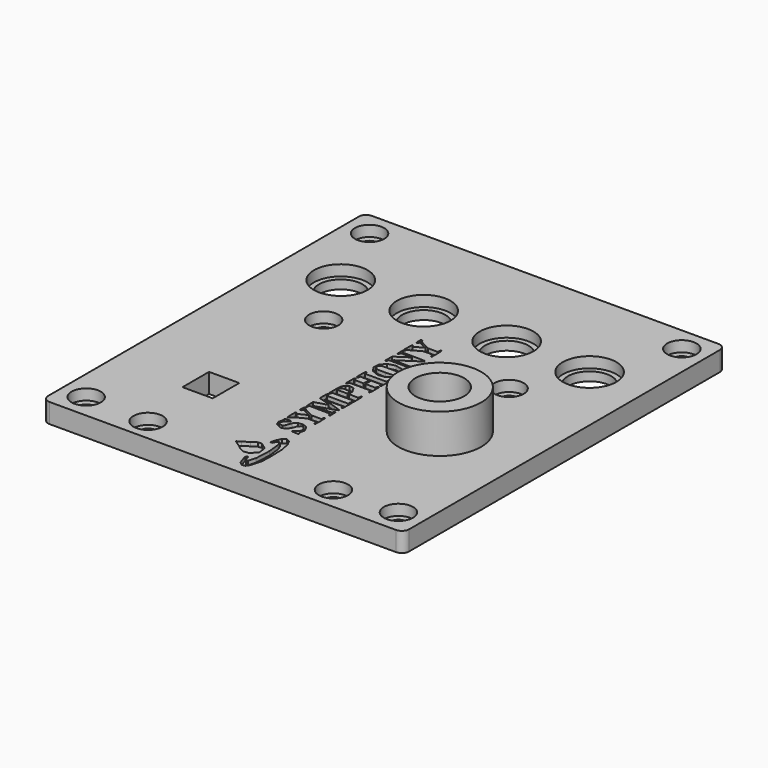
from build123d import *

# Parameters (mm, degrees)
F1_R      = 3
F1_R_2    = 1.75
F1_R_3    = 8.5
F1_R_4    = 0.9
F1_R_5    = 4.45
F1_R_6    = 1.7
F1_R_7    = 5
F1_W      = 7
F1_H      = 4.5
F2_DEPTH  = 4
F3_R      = 1.5
F4_R      = 3
F5_DEPTH  = 2.2
F6_R      = 5.5
F6_R_2    = 4.45
F7_DEPTH  = 2.2
F9_DEPTH  = 0.8
F10_R     = 5
F10_W     = 7
F10_H     = 4.5
F11_DEPTH = 2.1
F10_R_2   = 8.5
F12_DEPTH = 8
F13_W     = 6.2
F13_H     = 6.8
F14_DEPTH = 4


# Not quite as in the source:
# - ends of sketch curves that miss each other by under 0.0002 mm in the source are joined
# - a feature names something its author has since deleted; it is built from what else it names


with BuildPart() as f2:
    # F1 (on Top) → F2 (new body)
    with BuildSketch(Plane.XY):
        Polygon((-37, 10.5), (-37, -62.1), (37, -62.1), (37, 10.5), (37, 20.5), (-37, 20.5), align=None)
        with Locations((-32, -57.1)):
            Circle(F1_R, mode=Mode.SUBTRACT)
        with Locations((-19, -57.5)):
            Circle(F1_R_2, mode=Mode.SUBTRACT)
        with Locations((19, -57.5)):
            Circle(F1_R_2, mode=Mode.SUBTRACT)
        with Locations((32, -57.1)):
            Circle(F1_R, mode=Mode.SUBTRACT)
        with Locations((19.65, -31.075)):
            Circle(F1_R_3, mode=Mode.SUBTRACT)
        with Locations((-19, -12.5)):
            Circle(F1_R_2, mode=Mode.SUBTRACT)
        with Locations((-30.5, -5)):
            Circle(F1_R_4, mode=Mode.SUBTRACT)
        with Locations((-20.5, -5)):
            Circle(F1_R_4, mode=Mode.SUBTRACT)
        with Locations((-13.5, -5)):
            Circle(F1_R_4, mode=Mode.SUBTRACT)
        with Locations((-3.5, -5)):
            Circle(F1_R_4, mode=Mode.SUBTRACT)
        with Locations((-30.5, 5)):
            Circle(F1_R_4, mode=Mode.SUBTRACT)
        with Locations((-25.5, 0)):
            Circle(F1_R_5, mode=Mode.SUBTRACT)
        with Locations((-20.5, 5)):
            Circle(F1_R_4, mode=Mode.SUBTRACT)
        with Locations((-32, 15.5)):
            Circle(F1_R, mode=Mode.SUBTRACT)
        with Locations((-13.5, 5)):
            Circle(F1_R_4, mode=Mode.SUBTRACT)
        with Locations((-8.5, 0)):
            Circle(F1_R_5, mode=Mode.SUBTRACT)
        with Locations((-3.5, 5)):
            Circle(F1_R_4, mode=Mode.SUBTRACT)
        with Locations((3.5, -5)):
            Circle(F1_R_4, mode=Mode.SUBTRACT)
        with Locations((13.5, -5)):
            Circle(F1_R_4, mode=Mode.SUBTRACT)
        with Locations((19, -12.5)):
            Circle(F1_R_2, mode=Mode.SUBTRACT)
        with Locations((20.5, -5)):
            Circle(F1_R_4, mode=Mode.SUBTRACT)
        with Locations((30.5, -5)):
            Circle(F1_R_4, mode=Mode.SUBTRACT)
        with Locations((3.5, 5)):
            Circle(F1_R_4, mode=Mode.SUBTRACT)
        with Locations((8.5, 0)):
            Circle(F1_R_5, mode=Mode.SUBTRACT)
        with Locations((13.5, 5)):
            Circle(F1_R_4, mode=Mode.SUBTRACT)
        with Locations((20.5, 5)):
            Circle(F1_R_4, mode=Mode.SUBTRACT)
        with Locations((25.5, 0)):
            Circle(F1_R_5, mode=Mode.SUBTRACT)
        with Locations((30.5, 5)):
            Circle(F1_R_4, mode=Mode.SUBTRACT)
        with Locations((32, 15.5)):
            Circle(F1_R, mode=Mode.SUBTRACT)
        with Locations((-32, 15.5)):
            Circle(F1_R)
        with Locations((-32, 15.5)):
            Circle(F1_R_6, mode=Mode.SUBTRACT)
        with Locations((32, 15.5)):
            Circle(F1_R)
        with Locations((32, 15.5)):
            Circle(F1_R_6, mode=Mode.SUBTRACT)
        with Locations((-32, -57.1)):
            Circle(F1_R)
        with Locations((-32, -57.1)):
            Circle(F1_R_6, mode=Mode.SUBTRACT)
        with Locations((32, -57.1)):
            Circle(F1_R)
        with Locations((32, -57.1)):
            Circle(F1_R_6, mode=Mode.SUBTRACT)
        with Locations((-30.5, 5)):
            Circle(F1_R_4)
        with Locations((3.5, -5)):
            Circle(F1_R_4)
        with Locations((-30.5, -5)):
            Circle(F1_R_4)
        with Locations((-20.5, -5)):
            Circle(F1_R_4)
        with Locations((-13.5, -5)):
            Circle(F1_R_4)
        with Locations((-3.5, -5)):
            Circle(F1_R_4)
        with Locations((20.5, -5)):
            Circle(F1_R_4)
        with Locations((20.5, 5)):
            Circle(F1_R_4)
        with Locations((13.5, 5)):
            Circle(F1_R_4)
        with Locations((3.5, 5)):
            Circle(F1_R_4)
        with Locations((-20.5, 5)):
            Circle(F1_R_4)
        with Locations((13.5, -5)):
            Circle(F1_R_4)
        with Locations((-13.5, 5)):
            Circle(F1_R_4)
        with Locations((-3.5, 5)):
            Circle(F1_R_4)
        with Locations((30.5, 5)):
            Circle(F1_R_4)
        with Locations((30.5, -5)):
            Circle(F1_R_4)
        with Locations((19.65, -31.075)):
            Circle(F1_R_3)
        with Locations((19.65, -31.075)):
            Circle(F1_R_7, mode=Mode.SUBTRACT)
        with Locations((19.65, -31.075)):
            Circle(F1_R_7)
        with Locations((19.65, -31.075)):
            Rectangle(F1_W, F1_H, mode=Mode.SUBTRACT)
    extrude(amount=F2_DEPTH)

    # F3
    f3_edges = [f2.edges().sort_by_distance(p)[0] for p in [
        (-37, -62.1, 2),
        (37, -62.1, 2),
        (37, 20.5, 2),
        (-37, 20.5, 2),
    ]]
    fillet(f3_edges, radius=F3_R)

    # F4 (on face) → F5 (cut)
    with BuildSketch(Plane.XY.offset(4)):
        with Locations((-32, -57.1)):
            Circle(F4_R)
        with Locations((-32, 15.5)):
            Circle(F4_R)
        with Locations((32, 15.5)):
            Circle(F4_R)
        with Locations((32, -57.1)):
            Circle(F4_R)
        with Locations((-19, -57.5)):
            Circle(F4_R)
        with Locations((19, -57.5)):
            Circle(F4_R)
        with Locations((19, -12.5)):
            Circle(F4_R)
        with Locations((-19, -12.5)):
            Circle(F4_R)
    extrude(amount=-F5_DEPTH, mode=Mode.SUBTRACT)

    # F6 (on face) → F7 (cut)
    with BuildSketch(Plane.XY.offset(4)):
        with Locations((-25.5, 0)):
            Circle(F6_R)
        with Locations((-25.5, 0)):
            Circle(F6_R_2, mode=Mode.SUBTRACT)
        with Locations((-8.5, 0)):
            Circle(F6_R)
        with Locations((-8.5, 0)):
            Circle(F6_R_2, mode=Mode.SUBTRACT)
        with Locations((8.5, 0)):
            Circle(F6_R)
        with Locations((8.5, 0)):
            Circle(F6_R_2, mode=Mode.SUBTRACT)
        with Locations((25.5, 0)):
            Circle(F6_R)
        with Locations((25.5, 0)):
            Circle(F6_R_2, mode=Mode.SUBTRACT)
    extrude(amount=-F7_DEPTH, mode=Mode.SUBTRACT)

    # F8 (on face) → F9 (cut)
    with BuildSketch(Plane.XY.offset(4)):
        Polygon((3.3005577002, -59.0406586255), (3.8515091002, -57.0452346255), (3.8910315002, -56.7349736255), (3.9497055002, -54.5907564255), (3.8623549002, -51.6950802255), (3.4624827002, -49.7854066255), (2.8953769002, -48.7427366255), (2.2128789002, -48.4190898255), (1.5445287002, -48.8822080255), (1.1356141002, -49.7182490255), (0.8126785002, -50.8056738255), (0.8565443002, -50.9512158255), (1.0670849002, -50.4589892255), (1.4432081002, -49.4592706255), (1.9242333002, -48.9441078255), (2.4097289002, -49.0606176255), (2.8773175002, -49.8345048255), (3.4035039002, -52.3716854255), (3.4552183002, -55.0561860255), (3.0665475002, -57.9390606255), (2.5974857002, -59.0901378255), (2.1627647002, -59.4642290255), (1.7369337002, -59.3235384255), (1.2762031002, -58.5365448255), (0.9369607002, -57.5263360255), (0.8152439002, -57.3364964255), (0.8463843002, -57.6609306255), (1.4229643002, -59.3216842255), (2.1087135002, -59.9466512255), (2.7999999002, -59.7932860255), align=None)
        Polygon((1.0891321002, -57.0193266255), (0.8152439002, -57.3364964255), (0.9369607002, -57.5263360255), (1.2762031002, -58.5365448255), (1.7369337002, -59.3235384255), (2.1627647002, -59.4642290255), (2.5974857002, -59.0901378255), (3.0665475002, -57.9390606255), (3.4552183002, -55.0561860255), (3.4035039002, -52.3716854255), (2.8773175002, -49.8345048255), (2.4097289002, -49.0606176255), (1.9242333002, -48.9441078255), (1.4432081002, -49.4592706255), (1.0670849002, -50.4589892255), (0.8565443002, -50.9512158255), (1.2289337002, -50.8387192255), (1.1760509002, -50.6933550255), (1.4830099002, -49.9010274255), (1.8875811002, -49.5479928255), (2.3352561002, -49.7129912255), (2.7210821002, -50.5476352255), (3.0411729002, -53.2403654255), (2.9937257002, -56.1077206255), (2.9687067002, -56.3787894255), (2.5760227002, -58.0826976255), (2.1788429002, -58.6706060255), (1.9104919002, -58.7467552255), (1.4415571002, -58.2696670255), align=None)
        Polygon((1.1580677002, -57.0161516255), (1.0891321002, -57.0193266255), (1.4415571002, -58.2696670255), (1.9104919002, -58.7467552255), (2.1788429002, -58.6706060255), (2.5760227002, -58.0826976255), (2.9687067002, -56.3787894255), (2.9937257002, -56.1077206255), (3.0411729002, -53.2403654255), (2.7210821002, -50.5476352255), (2.3352561002, -49.7129912255), (1.8875811002, -49.5479928255), (1.4830099002, -49.9010274255), (1.1760509002, -50.6933550255), (1.2289337002, -50.8387192255), (1.5042951002, -50.2478898255), (1.7710205002, -49.9030340255), (2.0183403002, -50.0255128255), (2.3400821002, -50.8816960255), (2.6143767002, -53.3491790255), (2.4676155002, -56.6308590255), (2.0078501002, -58.2033222255), (1.7833141002, -58.3320494255), (1.4813335002, -57.9166070255), align=None)
        Polygon((1.2507523002, -45.8767784255), (2.5288295002, -45.8930344255), (2.6148593002, -45.8066998255), (2.3641359002, -45.3630380255), (2.4176029002, -45.0095208255), (2.5989589002, -44.2949934255), (1.9607585002, -43.1670048255), (1.0406689002, -42.8201678255), (0.0667313002, -42.9637794255), (-0.6000694998, -43.6390892255), (-1.0120320998, -44.8255232255), (-1.2610028998, -45.2329646255), (-2.1099978998, -44.9996910255), (-2.2472340998, -44.4760954255), (-2.0439578998, -43.9825226255), (-1.1984172998, -43.3929632255), (-1.1283132998, -43.1367534255), (-1.3950132998, -43.0616456255), (-2.2405792998, -43.0750314255), (-2.5238400998, -43.2081782255), (-2.4127404998, -43.5266688255), (-2.4304442998, -43.8971532255), (-2.6180740998, -44.4731490255), (-2.3431698998, -45.3219408255), (-1.0647878998, -45.9625034255), (-0.1445204998, -45.6985212255), (0.4974391002, -44.7151602255), (0.6744009002, -44.1188190255), (1.1787687002, -43.4875528255), (1.7564155002, -43.5680708255), (2.2070877002, -44.1221210255), (2.0958103002, -44.8600418255), (1.5639089002, -45.3874982255), (1.2146335002, -45.5068528255), (1.0236509002, -45.7635452255), align=None)
        Polygon((1.1297467002, -21.7921936255), (2.4470923002, -20.5285182255), (2.5894593002, -20.0451562255), (2.3140471002, -18.8252196255), (1.3973865002, -17.9522470255), (-0.0992068998, -17.6598422255), (-1.6222670998, -18.0603494255), (-2.4897278998, -19.1916654255), (-2.5484526998, -20.3214574255), (-1.7673010998, -21.4095172255), (-0.3714694998, -21.9864782255), align=None)
        Polygon((1.7325395002, -19.1622014255), (2.0332755002, -19.3513806255), (2.1802399002, -19.5659598255), (2.0936259002, -20.2633930255), (1.5780059002, -20.4864812255), (0.0999545002, -20.5732984255), (-1.4272458998, -20.5208474255), (-1.9467520998, -20.3856432255), (-2.2429160998, -19.9628602255), (-2.1648618998, -19.4758660255), (-1.8558200998, -19.1899636255), (-1.2080946998, -19.1180054255), (0.8853479002, -19.1136366255), align=None, mode=Mode.SUBTRACT)
        Polygon((-1.5965114998, -16.4241068255), (0.5155239002, -15.0651814255), (1.8799865002, -14.1600270255), (2.5557281002, -13.6388190255), (2.4666249002, -13.4825836255), (1.6060983002, -13.4359746255), (-1.6538392998, -13.4149942255), (-2.1118520998, -13.3087206255), (-2.2307240998, -12.9749900255), (-2.4305204998, -12.8264254255), (-2.5017674998, -13.0967068255), (-2.5028850998, -14.0661486255), (-2.4309268998, -14.3534480255), (-2.2293016998, -14.2101158255), (-2.1485550998, -13.7854786255), (-2.0495966998, -13.7832180255), (-0.4457390998, -13.7528650255), (0.1292153002, -13.7842848255), (-0.0456890998, -13.9309698255), (-2.5134768998, -15.5511850255), (-2.5340000998, -16.3011454255), (-2.5415946998, -17.2603002255), (-2.4113688998, -17.4494032255), (-2.2063908998, -17.3136910255), (-2.1954434998, -16.8638570255), (2.1533667002, -16.8638570255), (2.2075449002, -17.2541534255), (2.4080017002, -17.3741430255), (2.4877323002, -17.0290332255), (2.5183901002, -16.0558830255), (2.4524263002, -15.8085886255), (2.2034301002, -15.8496096255), (2.1485407002, -16.2454178255), (2.0111267002, -16.4363242255), (0.9230923002, -16.4574316255), align=None)
        Polygon((2.2163587002, -41.4657890255), (2.4405137002, -41.5374932255), (2.4761499002, -41.4328960255), (2.5123703002, -40.4028244255), (2.4668027002, -39.0928702255), (2.3857513002, -38.8148164255), (2.2070115002, -38.9910416255), (2.1544843002, -39.5358716255), (0.1212905002, -39.5376242255), (-0.4593280998, -39.2467434255), (-1.7954442998, -38.5486752255), (-2.1526952998, -38.2283050255), (-2.3678078998, -37.9732890255), (-2.5377084998, -38.1173832255), (-2.5577236998, -38.7984080255), (-2.5063140998, -39.1919810255), (-2.2664364998, -39.2151712255), (-2.1745900998, -38.9091774255), (-1.9572422998, -38.9149432255), (-0.2584902998, -39.7212662255), (-0.7021520998, -39.9445830255), (-1.8695360998, -40.5224076255), (-2.1379886998, -40.5765604255), (-2.2115216998, -40.3276912255), (-2.4845970998, -40.2466398255), (-2.5457602998, -40.5277162255), (-2.5283104998, -41.7582700255), (-2.4662074998, -42.4220990255), (-2.2525172998, -42.4283982255), (-2.1099470998, -42.1614188255), (-1.3831006998, -41.6910870255), (0.2592633002, -40.8062526255), (2.1549415002, -40.8062526255), (2.1654317002, -40.8903520255), align=None)
        Polygon((2.1680987002, -37.5476866255), (2.3741943002, -37.8568046255), (2.4756165002, -37.8357734255), (2.5188981002, -37.5539604255), (2.4830079002, -36.5044324255), (2.4011691002, -36.1851544255), (2.1991883002, -36.3260736255), (2.1183401002, -36.7507108255), (-1.6049188998, -36.7883028255), (-0.0626562998, -36.3049408255), (1.6711985002, -35.7591456255), (2.4721113002, -35.4356258255), (2.4242831002, -35.3210210255), (1.1269019002, -34.8458886255), (-1.3416732998, -34.0745668255), (-1.4984674998, -34.0201346255), (-0.5653730998, -33.9857176255), (2.1539255002, -33.9655500255), (2.1809765002, -34.2674798255), (2.3010677002, -34.5888914255), (2.4553727002, -34.4121582255), (2.5085857002, -33.3668212255), (2.5084587002, -32.3154898255), (2.3810777002, -32.1096482255), (2.1763791002, -32.2454366255), (2.1654317002, -32.6951436255), (-2.1954688998, -32.6951436255), (-2.1954688998, -32.4492462255), (-2.2575718998, -32.1414490255), (-2.4944268998, -32.1516344255), (-2.5535834998, -32.5223474255), (-2.5588666998, -34.0557454255), (-1.1746428998, -34.4788332255), (-0.1651706998, -34.7993050255), (-0.0150312998, -34.9607474255), (-0.4846010998, -35.1421034255), (-2.5648102998, -35.7486046255), (-2.5529992998, -36.2251848255), (-2.5042820998, -37.5254362255), (-2.4235100998, -37.8097892255), (-2.2371502998, -37.6572622255), (-2.1836832998, -37.1869558255), (2.1183147002, -37.2393052255), align=None)
        Polygon((2.2197877002, -31.9054830255), (2.4406407002, -31.9604486255), (2.4741433002, -31.8721582255), (2.5133609002, -31.0791448255), (2.4725939002, -29.7515884255), (2.3939809002, -29.4393970255), (2.2078751002, -29.5989090255), (2.1575069002, -30.1054612255), (0.2244145002, -30.0461776255), (0.1665025002, -30.0050042255), (0.1178107002, -29.0488466255), (-0.5257998998, -27.9611170255), (-1.4718228998, -27.8132636255), (-2.0676052998, -28.1399330255), (-2.4260500998, -28.7757204255), (-2.5122068998, -30.0546612255), (-2.4937410998, -31.6093698255), (-2.4246276998, -31.9415002255), (-2.2284380998, -31.8012922255), (-2.1500282998, -31.3758676255), (2.1077229002, -31.3758676255), (2.1655079002, -31.4129516255), align=None)
        Polygon((-0.7558476998, -29.1257578255), (-0.3256478998, -29.2896894255), (-0.2993588998, -29.3231158255), (-0.0831540998, -30.0565916255), (-2.1113948998, -30.0565916255), (-2.1954434998, -30.0435868255), (-2.1593500998, -29.5278906255), (-1.7056044998, -29.1465350255), align=None, mode=Mode.SUBTRACT)
        Polygon((2.1718579002, -27.3498914255), (2.3471433002, -27.5157788255), (2.3627897002, -27.5155502255), (2.5046741002, -27.3231452255), (2.5288295002, -26.3344248255), (2.5067315002, -25.2816710255), (2.3775217002, -25.0736958255), (2.1763791002, -25.2099160255), (2.1654571002, -25.6590134255), (0.0758499002, -25.6590134255), (0.0758499002, -24.1931540255), (2.1654571002, -24.1931540255), (2.1739661002, -24.6283322255), (2.3628151002, -24.7792844255), (2.5046995002, -24.5868794255), (2.5288549002, -23.5981590255), (2.5067569002, -22.5454052255), (2.3775471002, -22.3374046255), (2.1763791002, -22.4736502255), (2.1654571002, -22.9227476255), (-2.1954180998, -22.9227476255), (-2.2039524998, -22.4875694255), (-2.3927760998, -22.3366172255), (-2.5346604998, -22.5290222255), (-2.5588158998, -23.5177426255), (-2.5367178998, -24.5704964255), (-2.4075080998, -24.7784970255), (-2.2063654998, -24.6422514255), (-2.1954434998, -24.1931540255), (-0.2875478998, -24.1931540255), (-0.2875478998, -25.6590134255), (-2.1954434998, -25.6590134255), (-2.2039524998, -25.2238352255), (-2.3928014998, -25.0729084255), (-2.5346858998, -25.2653134255), (-2.5588412998, -26.2540084255), (-2.5367432998, -27.3067622255), (-2.4075334998, -27.5147628255), (-2.2063908998, -27.3785172255), (-2.1954688998, -26.9294198255), (2.1654317002, -26.9294198255), align=None)
        Polygon((2.2379487002, -11.6438776255), (2.4769881002, -11.7076824255), (2.4903485002, -11.6505578255), (2.5124719002, -10.5891934255), (2.4667519002, -9.2847256255), (2.3857259002, -9.0088308255), (2.2069861002, -9.1851322255), (2.1544589002, -9.7299876255), (0.1616511002, -9.7299876255), (-1.1645590998, -9.0691812255), (-2.0029876998, -8.5843206255), (-2.1956466998, -8.2383218255), (-2.4062888998, -8.0695642255), (-2.5431948998, -8.2518092255), (-2.5561742998, -9.0456862255), (-2.4998116998, -9.3938694255), (-2.2529490998, -9.3994066255), (-2.1583340998, -9.0794174255), (-1.9138082998, -9.1165522255), (-0.2684724998, -9.8703226255), (-2.0850296998, -10.8330588255), (-2.1544224998, -10.8436506255), (-2.2454052998, -10.4761888255), (-2.4538122998, -10.4262778255), (-2.5206142998, -10.9375544255), (-2.5480970998, -12.2911712255), (-2.4918106998, -12.6276196255), (-2.2330862998, -12.6043024255), (-2.1092612998, -12.3554332255), (-1.3763188998, -11.8816724255), (0.2592633002, -11.0004194255), (2.1549415002, -11.0004194255), (2.1654317002, -11.0850776255), align=None)
        Polygon((0.5062021002, -55.9696716255), (1.6147851002, -54.7319042255), (1.4155729002, -53.1233984255), (0.0049585002, -52.1134944255), (-0.7279838998, -52.1670630255), (-1.7774356998, -52.8210876255), (-2.9215532998, -53.6390438255), (-3.5180976998, -53.9542832255), (-3.7363090998, -54.1031272255), (-3.4573154998, -54.3033300255), (-2.7790338998, -54.7375684255), (-1.5802300998, -55.6260350255), (-0.6610040998, -56.1159248255), align=None)
    extrude(amount=-F9_DEPTH, mode=Mode.SUBTRACT)

    # F10 (on face) → F11 (cut)
    with BuildSketch(Plane.XY.offset(4)):
        with Locations((19.65, -31.075)):
            Circle(F10_R)
        with Locations((19.65, -31.075)):
            Rectangle(F10_W, F10_H, mode=Mode.SUBTRACT)
    extrude(amount=-F11_DEPTH, mode=Mode.SUBTRACT)

    # F10 (on face) → F12 (join)
    with BuildSketch(Plane.XY.offset(4)):
        with Locations((19.65, -31.075)):
            Circle(F10_R_2)
        with Locations((19.65, -31.075)):
            Circle(F10_R, mode=Mode.SUBTRACT)
    extrude(amount=F12_DEPTH)

    # F13 (on face) → F14 (cut)
    with BuildSketch(Plane.XY.offset(4)):
        with Locations((-19, -41.4)):
            Rectangle(F13_W, F13_H)
    extrude(amount=-F14_DEPTH, mode=Mode.SUBTRACT)


solid = f2.part
